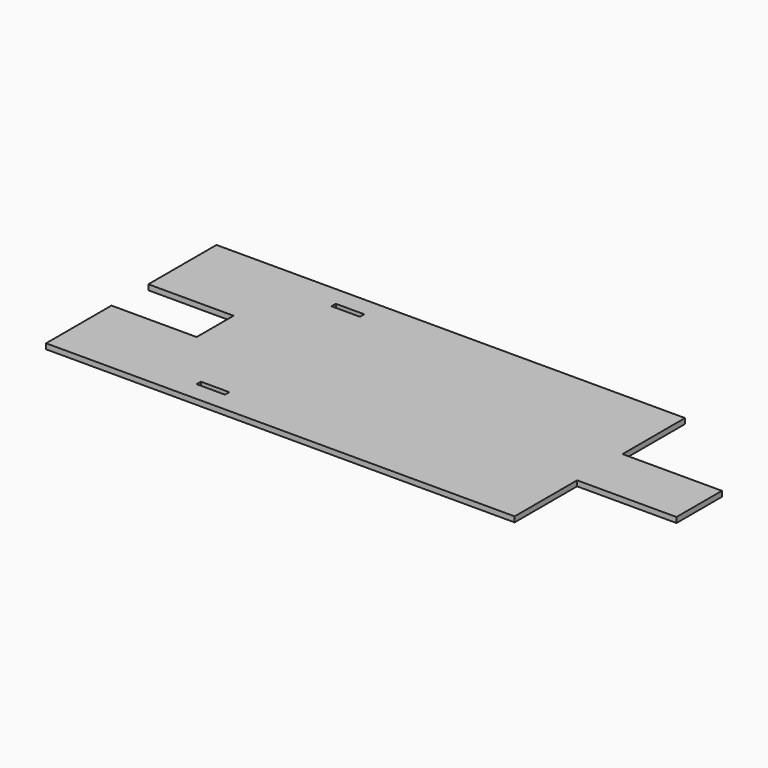
from build123d import *

# Parameters (mm, degrees)
F1_DEPTH = 19.05
F2_W     = 101.854
F2_H     = 19.304
F3_DEPTH = 25.4


# Not quite as in the source:
# - a feature names something its author has since deleted; it is built from what else it names


with BuildPart() as f1:
    # F0 (on Top) → F1 (new body)
    with BuildSketch(Plane.XY):
        Polygon((-69.3041831255, 0), (-69.3041831255, -150.0828219056), (1607.0958168745, -150.0828219056), (1607.0958168745, 129.3171780944), (1962.6958168745, 129.3171780944), (1962.6958168745, 332.5171780944), (1607.0958168745, 332.5171780944), (1607.0958168745, 611.9171780944), (-69.3041831255, 611.9171780944), align=None)
    extrude(amount=F1_DEPTH)

    # F2 (on face) → F3 (cut)
    with BuildSketch(Plane.XY.offset(19.05)):
        with Locations((464.2228168745, 532.6691780944)):
            Rectangle(F2_W, F2_H)
        with Locations((464.2228168745, -70.8348219056)):
            Rectangle(F2_W, F2_H)
        Polygon((-69.3041831255, 307.3549188137), (-69.3041831255, 224.8049188137), (-69.3041831255, 142.2549188137), (235.4958168745, 142.2549188137), (235.4958168745, 307.3549188137), align=None)
    extrude(amount=-F3_DEPTH, mode=Mode.SUBTRACT)


solid = f1.part
